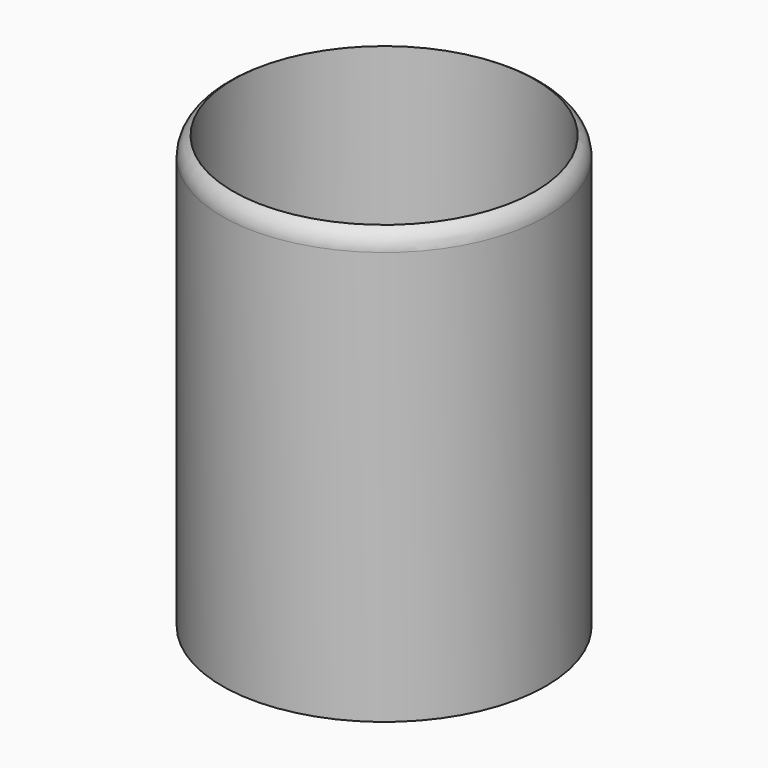
from build123d import *

# Parameters (mm, degrees)
F0_R     = 38.1
F1_DEPTH = 101.6
F2_T     = -2.54


# Not quite as in the source:
# - a fillet or chamfer that OpenCascade refuses, or shapes differently, is made with other operations: its cross-section is extruded or revolved along the edge and cut away or added


with BuildPart() as f1:
    # F0 (on Top) → F1 (new body)
    with BuildSketch(Plane.XY):
        Circle(F0_R)
    extrude(amount=F1_DEPTH)

    # F2
    f2_openings = [f1.faces().sort_by_distance(p)[0] for p in [
        (0, 0, 101.6),
    ]]
    offset(amount=F2_T, openings=f2_openings)

    # F3: fillet of radius 5.08 on 1 edges, made by hand

    # F3_s1 → F3_t2 (revolve, cut)
    with BuildSketch(Plane.XZ):
        with BuildLine():
            ThreePointArc((38.1, 97.2005909488), (37.4194090512, 99.7405909488), (35.56, 101.6))
            Line((35.56, 101.6), (38.1, 101.6))
            Line((38.1, 101.6), (38.1, 97.2005909488))
        make_face()
    revolve(axis=Axis((0, 0, 101.6), (0, 0, 1)), mode=Mode.SUBTRACT)


solid = f1.part
